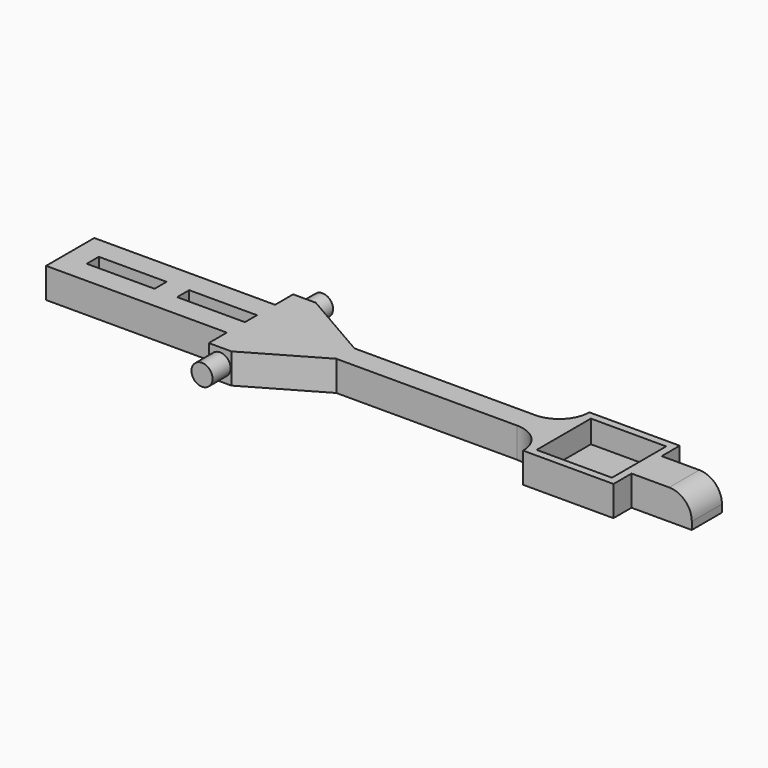
from build123d import *

# Parameters (mm, degrees)
F0_W     = 28.575
F0_H     = 6.35
F1_DEPTH = 12.7
F2_R     = 4.445
F3_DEPTH = 9.525
F4_R     = 4.445
F5_DEPTH = 9.525
F6_W     = 31.75
F6_H     = 28.575
F7_DEPTH = 9.525
F8_R     = 9.52499


# Not quite as in the source:
# - a fillet or chamfer is up to 0.001 mm smaller than in the source, because OpenCascade refuses the exact size


with BuildPart() as f1:
    # F0 (on Top) → F1 (new body)
    with BuildSketch(Plane.XY):
        with BuildLine():
            Line((-76.2, -12.7), (0, -12.7))
            Line((0, -12.7), (0, -22.225))
            Line((0, -22.225), (9.525, -22.225))
            Line((9.525, -22.225), (39.7709372272, -4.7625))
            Line((39.7709372272, -4.7625), (115.9709372272, -4.7625))
            ThreePointArc((115.9709372272, -4.7625), (124.9511933482, -8.4822438789), (128.6709372272, -17.4625))
            Line((128.6709372272, -17.4625), (166.7709372272, -17.4625))
            Line((166.7709372272, -17.4625), (166.7709372272, -7.9375))
            Line((166.7709372272, -7.9375), (192.1709372272, -7.9375))
            Line((192.1709372272, -7.9375), (192.1709372272, 7.9375))
            Line((192.1709372272, 7.9375), (166.7709372272, 7.9375))
            Line((166.7709372272, 7.9375), (166.7709372272, 17.4625))
            Line((166.7709372272, 17.4625), (128.6709372272, 17.4625))
            ThreePointArc((128.6709372272, 17.4625), (124.9511933482, 8.4822438789), (115.9709372272, 4.7625))
            Line((115.9709372272, 4.7625), (39.7709372272, 4.7625))
            Line((39.7709372272, 4.7625), (9.525, 22.225))
            Line((9.525, 22.225), (0, 22.225))
            Line((0, 22.225), (0, 12.7))
            Line((0, 12.7), (-76.2, 12.7))
            Line((-76.2, 12.7), (-76.2, -12.7))
        make_face()
        with Locations((-52.3875, 0)):
            Rectangle(F0_W, F0_H, mode=Mode.SUBTRACT)
        with Locations((-14.2875, 0)):
            Rectangle(F0_W, F0_H, mode=Mode.SUBTRACT)
    extrude(amount=F1_DEPTH)

    # F2 (on face) → F3 (join)
    with BuildSketch(Plane.XZ.offset(22.225)):
        with Locations((4.7625, 6.35)):
            Circle(F2_R)
    extrude(amount=F3_DEPTH)

    # F4 (on face) → F5 (join)
    with BuildSketch(Plane(origin=(0, 22.225, 0), x_dir=(-1, 0, 0), z_dir=(0, 1, 0))):
        with Locations((-4.7625, 6.35)):
            Circle(F4_R)
    extrude(amount=F5_DEPTH)

    # F6 (on face) → F7 (cut)
    with BuildSketch(Plane.XY.offset(12.7)):
        with Locations((147.7209372272, 0)):
            Rectangle(F6_W, F6_H)
    extrude(amount=-F7_DEPTH, mode=Mode.SUBTRACT)

    # F8 (radius 9.525 in the source; OpenCascade refuses exactly that, so slightly less here)
    f8_edges = [f1.edges().sort_by_distance(p)[0] for p in [
        (163.595937, 0, 3.175),
        (192.170937, 0, 12.7),
    ]]
    fillet(f8_edges, radius=F8_R)


solid = f1.part
